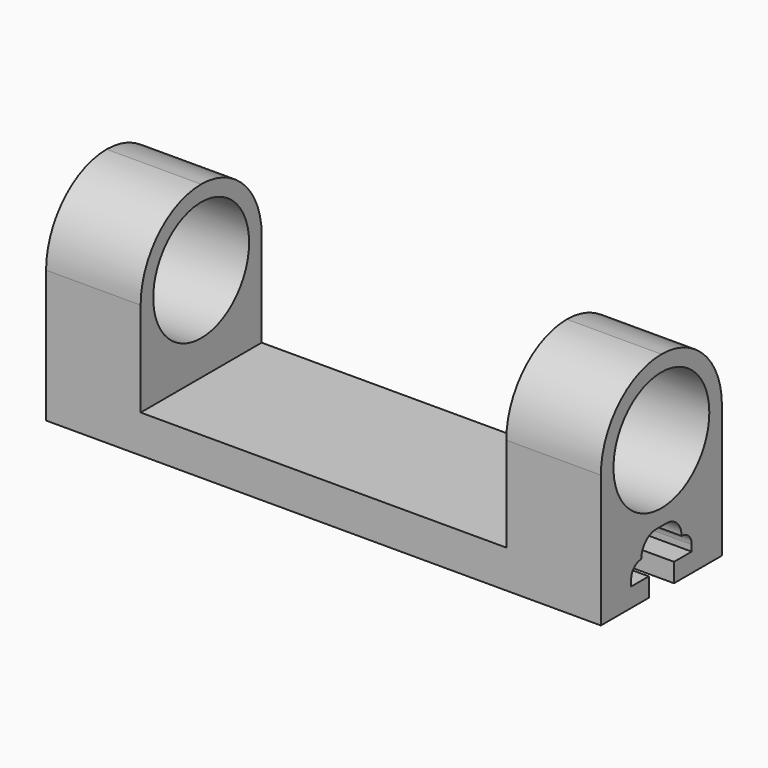
from build123d import *

# Parameters (mm, degrees)
F0_R     = 9.5
F1_DEPTH = 88
F2_W     = 58
F2_H     = 27
F3_DEPTH = 12.5
F4_DEPTH = 10
F6_DEPTH = 10
F7_R     = 2.99999
F8_R     = 1.99999


# Not quite as in the source:
# - a fillet or chamfer is up to 0.001 mm smaller than in the source, because OpenCascade refuses the exact size


with BuildPart() as f1:
    # F0 (on Right) → F1 (new body)
    with BuildSketch(Plane.YZ):
        with BuildLine():
            ThreePointArc((0, 9), (-8.4852813742, 12.5147186258), (-12, 21))
            Line((-12, 21), (-12, 0))
            Line((-12, 0), (-2.5, 0))
            Line((-2.5, 0), (-2.5, 3))
            Line((-2.5, 3), (-6, 3))
            Line((-6, 3), (-6, 6))
            Line((-6, 6), (-4, 6))
            Line((-4, 6), (-4, 9))
            Line((-4, 9), (0, 9))
        make_face()
        Polygon((4, 9), (0, 9), (-4, 9), (-4, 6), (-6, 6), (-6, 3), (-2.5, 3), (-2.5, 0), (2.5, 0), (2.5, 3), (6, 3), (6, 6), (4, 6), align=None)
        with BuildLine():
            Line((12, 0), (12, 21))
            ThreePointArc((12, 21), (8.4852813742, 12.5147186258), (0, 9))
            Line((0, 9), (4, 9))
            Line((4, 9), (4, 6))
            Line((4, 6), (6, 6))
            Line((6, 6), (6, 3))
            Line((6, 3), (2.5, 3))
            Line((2.5, 3), (2.5, 0))
            Line((2.5, 0), (12, 0))
        make_face()
        with BuildLine():
            ThreePointArc((12, 21), (8.4852813742, 29.4852813742), (0, 33))
            ThreePointArc((0, 33), (-8.4852813742, 29.4852813742), (-12, 21))
            ThreePointArc((-12, 21), (-8.4852813742, 12.5147186258), (0, 9))
            ThreePointArc((0, 9), (8.4852813742, 12.5147186258), (12, 21))
        make_face()
        with Locations((0, 21)):
            Circle(F0_R, mode=Mode.SUBTRACT)
    extrude(amount=-F1_DEPTH)

    # F2 (on Front) → F3 (cut, symmetric)
    with BuildSketch(Plane.XZ):
        with Locations((-44, 19.5)):
            Rectangle(F2_W, F2_H)
    extrude(amount=F3_DEPTH, both=True, mode=Mode.SUBTRACT)

    # F0 (on Right) → F4 (cut)
    with BuildSketch(Plane.YZ):
        Polygon((4, 9), (0, 9), (-4, 9), (-4, 6), (-6, 6), (-6, 3), (-2.5, 3), (-2.5, 0), (2.5, 0), (2.5, 3), (6, 3), (6, 6), (4, 6), align=None)
    extrude(amount=-F4_DEPTH, mode=Mode.SUBTRACT)

    # F5 (on face) → F6 (cut)
    with BuildSketch(Plane(origin=(-88, 0, 0), x_dir=(0, -1, 0), z_dir=(-1, 0, 0))):
        Polygon((-2.5, 3), (-2.5, 0), (2.5, 0), (2.5, 3), (6, 3), (6, 6), (4, 6), (4, 9), (0, 9), (-4, 9), (-4, 6), (-6, 6), (-6, 3), align=None)
    extrude(amount=-F6_DEPTH, mode=Mode.SUBTRACT)

    # F7 (radius 3 in the source; OpenCascade refuses exactly that, so slightly less here)
    f7_edges = [f1.edges().sort_by_distance(p)[0] for p in [
        (-83, 4, 9),
        (-83, -4, 9),
        (-5, -4, 9),
        (-5, 4, 9),
    ]]
    fillet(f7_edges, radius=F7_R)

    # F8 (radius 2 in the source; OpenCascade refuses exactly that, so slightly less here)
    f8_edges = [f1.edges().sort_by_distance(p)[0] for p in [
        (-83, -6, 6),
        (-83, 6, 6),
        (-5, 6, 6),
        (-5, -6, 6),
    ]]
    fillet(f8_edges, radius=F8_R)


solid = f1.part
